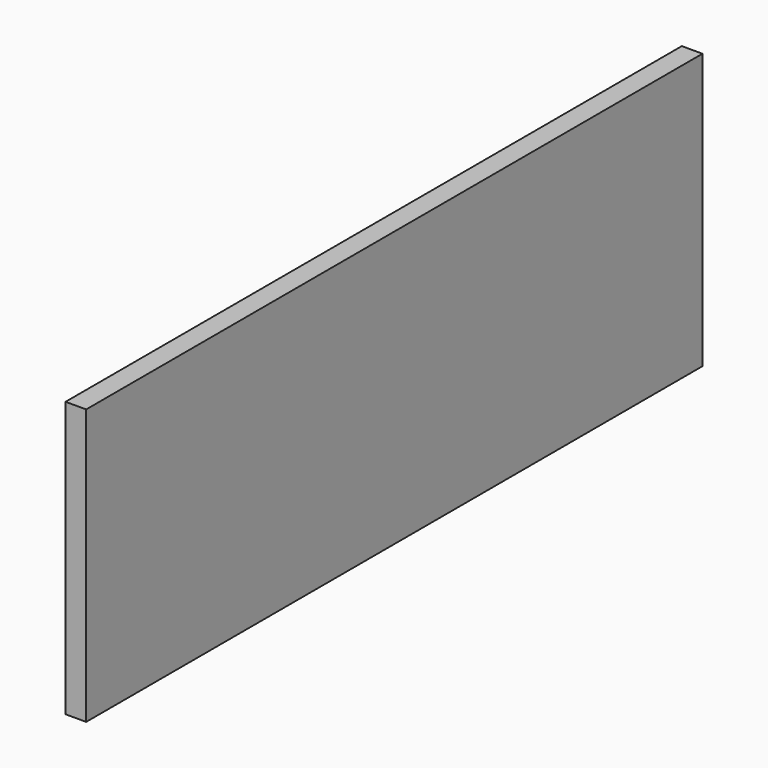
from build123d import *

# Parameters (mm, degrees)
F0_W     = 560
F0_H     = 200
F1_DEPTH = 7.5


with BuildPart() as f1:
    # F0 (on Right) → F1 (new body, symmetric)
    with BuildSketch(Plane.YZ):
        Rectangle(F0_W, F0_H)
    extrude(amount=F1_DEPTH, both=True)


solid = f1.part
